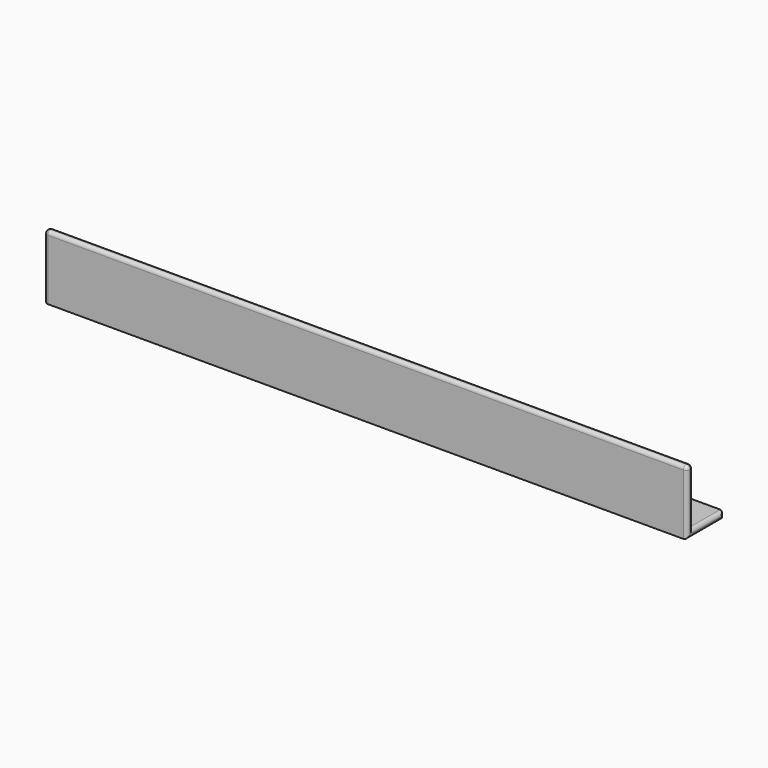
from build123d import *

# Parameters (mm, degrees)
F1_DEPTH = 88.9
F2_R     = 0.99999


# Not quite as in the source:
# - a fillet or chamfer is up to 0.001 mm smaller than in the source, because OpenCascade refuses the exact size


with BuildPart() as f1:
    # F0 (on Right) → F1 (new body, symmetric)
    with BuildSketch(Plane.YZ):
        Polygon((0, 17.78), (0, 0), (12.7, 0), (12.7, 2), (2, 2), (2, 17.78), align=None)
    extrude(amount=F1_DEPTH, both=True)

    # F2 (radius 1 in the source; OpenCascade refuses exactly that, so slightly less here)
    f2_edges = [f1.edges().sort_by_distance(p)[0] for p in [
        (0, 0, 17.78),
        (88.9, 0, 8.89),
        (-88.9, 1, 17.78),
        (88.9, 1, 17.78),
        (0, 2, 17.78),
        (88.9, 2, 9.89),
        (88.9, 6.35, 0),
        (88.9, 12.7, 1),
        (88.9, 7.35, 2),
        (-88.9, 0, 8.89),
        (-88.9, 2, 9.89),
        (-88.9, 7.35, 2),
        (-88.9, 6.35, 0),
    ]]
    fillet(f2_edges, radius=F2_R)


solid = f1.part
